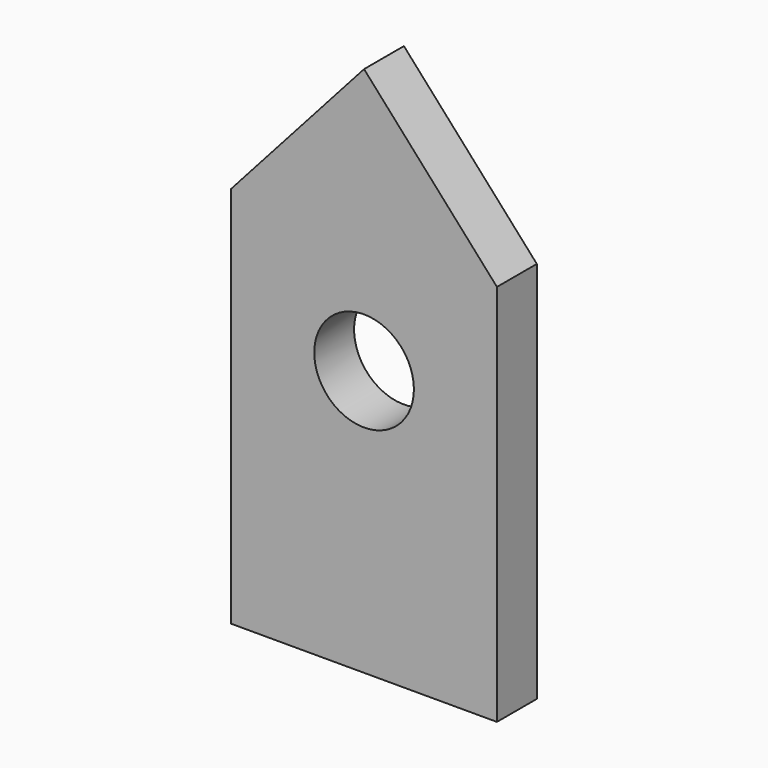
from build123d import *

# Parameters (mm, degrees)
F0_W     = 101.6
F0_H     = 203.2
F1_DEPTH = 19.05
F3_DEPTH = 19.051
F4_R     = 19.05
F5_DEPTH = 19.051


# Not quite as in the source:
# - a feature names something its author has since deleted; it is built from what else it names


with BuildPart() as f1:
    # F0 (on Front) → F1 (new body)
    with BuildSketch(Plane.XZ):
        Rectangle(F0_W, F0_H)
    extrude(amount=F1_DEPTH)

    # F2 (on face) → F3 (cut, through all)
    with BuildSketch(Plane.XZ.offset(19.05)):
        Polygon((-50.8, 44.8038733715), (0, 101.6), (-50.8, 101.6), align=None)
        Polygon((50.8, 101.6), (0, 101.6), (50.8, 44.8038733715), align=None)
    extrude(amount=-F3_DEPTH, mode=Mode.SUBTRACT)

    # F4 (on face) → F5 (cut, through all)
    with BuildSketch(Plane.XZ.offset(19.05)):
        Circle(F4_R)
    extrude(amount=-F5_DEPTH, mode=Mode.SUBTRACT)


solid = f1.part
